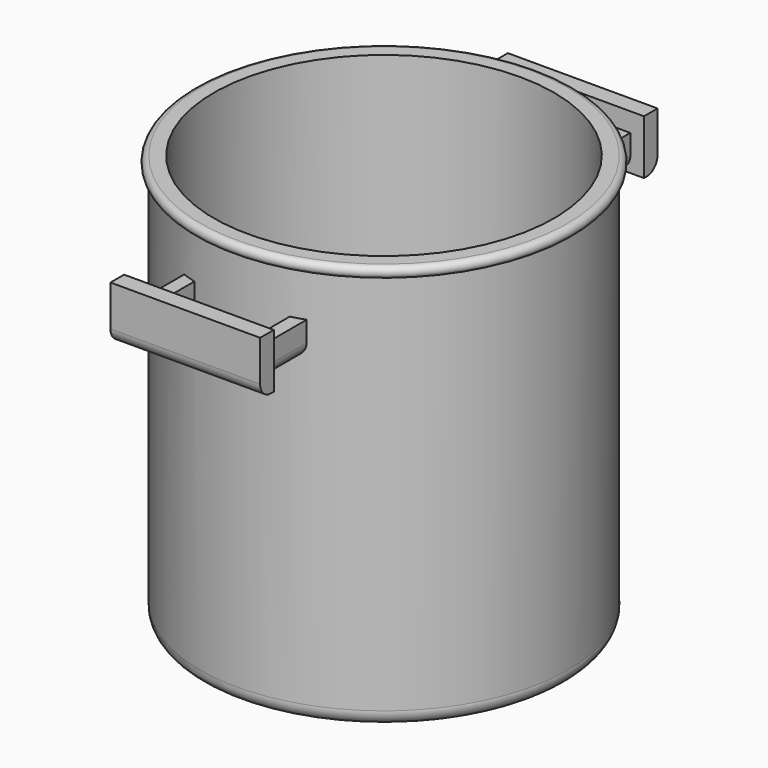
from build123d import *

# Parameters (mm, degrees)
F3_W      = 5.08
F3_H      = 12.7
F6_W      = 55.88
F6_H      = 20.32
F7_DEPTH  = 6.35
F10_W     = 5.08
F10_H     = 12.7
F12_W     = 55.88
F12_H     = 20.32
F13_DEPTH = 6.35
F14_R     = 5.08
F15_R     = 5.08
F16_R     = 5.07999


# Not quite as in the source:
# - a fillet or chamfer is up to 0.001 mm smaller than in the source, because OpenCascade refuses the exact size


with BuildPart() as f1:
    # F0 (on Right) → F1 (revolve)
    with BuildSketch(Plane.YZ):
        with BuildLine():
            Line((63.5, 5.08), (0, 5.08))
            Line((0, 5.08), (0, 0))
            Line((0, 0), (63.3201003075, 0))
            ThreePointArc((63.3201003075, 0), (67.2357467781, 1.5686265864), (68.58, 5.5668586865))
            Line((68.58, 5.5668586865), (68.58, 148.1529325247))
            ThreePointArc((68.58, 148.1529325247), (70.7035337377, 150.2764662623), (68.58, 152.4))
            Line((68.58, 152.4), (63.5, 152.4))
            Line((63.5, 152.4), (63.5, 5.08))
        make_face()
    revolve(axis=Axis((0, 0, 2.54), (0, 0, 1)))

    # F3 (on offset) → F4 (join, up to the next surface of F1)
    with BuildSketch(Plane.XZ.offset(86.36)):
        with Locations((-20.32, 125.8009325247)):
            Rectangle(F3_W, F3_H)
        with Locations((20.32, 125.8009325247)):
            Rectangle(F3_W, F3_H)
    extrude(until=Until.NEXT, dir=(0, 1, 0))

    # F6 (on offset) → F7 (join, through all)
    with BuildSketch(Plane.XZ.offset(92.71)):
        with Locations((0, 129.1029325247)):
            Rectangle(F6_W, F6_H)
    extrude(amount=-F7_DEPTH)

    # F10 (on offset) → F11 (join, up to the next surface of F1)
    with BuildSketch(Plane.XZ.offset(-86.36)):
        with Locations((20.32, 125.8009325247)):
            Rectangle(F10_W, F10_H)
        with Locations((-20.32, 125.8009325247)):
            Rectangle(F10_W, F10_H)
    extrude(until=Until.NEXT)

    # F12 (on offset) → F13 (join, through all)
    with BuildSketch(Plane.XZ.offset(-92.71)):
        with Locations((0, 129.1029325247)):
            Rectangle(F12_W, F12_H)
    extrude(amount=F13_DEPTH)

    # F14
    f14_edges = [f1.edges().sort_by_distance(p)[0] for p in [
        (0, -92.71, 118.942933),
    ]]
    fillet(f14_edges, radius=F14_R)

    # F15
    f15_edges = [f1.edges().sort_by_distance(p)[0] for p in [
        (0, 92.71, 118.942933),
    ]]
    fillet(f15_edges, radius=F15_R)

    # F16 (radius 5.08 in the source; OpenCascade refuses exactly that, so slightly less here)
    f16_edges = [f1.edges().sort_by_distance(p)[0] for p in [
        (-22.86, 75.508922, 119.450933),
        (22.86, 75.508922, 119.450933),
        (-22.86, -75.508922, 119.450933),
        (22.86, -75.508922, 119.450933),
    ]]
    fillet(f16_edges, radius=F16_R)


solid = f1.part
